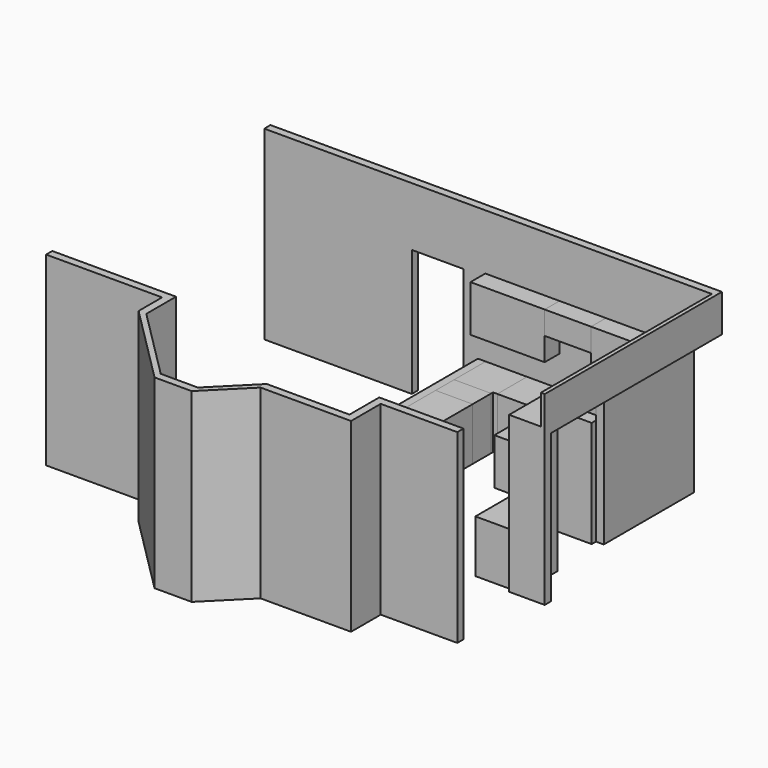
from build123d import *

# Parameters (mm, degrees)
F0_W      = 3556
F0_H      = 127
F1_DEPTH  = 3048
F3_DEPTH  = 3048
F4_W      = 127
F4_H      = 838.2
F5_DEPTH  = 3048
F6_W      = 1016
F6_H      = 127
F7_DEPTH  = 3048
F8_W      = 127
F8_H      = 482.6
F9_DEPTH  = 3048
F10_W     = 368.3
F10_H     = 127
F11_DEPTH = 3048
F12_W     = 996.95
F12_H     = 2095.5
F13_DEPTH = 25.4
F14_W     = 850.9
F14_H     = 965.2
F15_DEPTH = 127
F16_W     = 127
F16_H     = 965.2
F16_H_2   = 2082.8
F17_DEPTH = 2423.611736456
F18_W     = 1059.5979121052
F18_H     = 933.45
F19_DEPTH = 127
F21_W     = 457.2
F21_H     = 127
F22_DEPTH = 3048
F24_W     = 520.7
F24_H     = 3638.55
F25_DEPTH = 127
F26_W     = 3699.2286321938
F26_H     = 1626.0209083557
F27_DEPTH = 1270
F29_DEPTH = 127
F30_W     = 63.5
F30_H     = 615.95
F31_DEPTH = 3511.55
F32_W     = 685.8
F32_H     = 863.6
F33_DEPTH = 609.6
F34_W     = 685.8
F34_H     = 762
F35_DEPTH = 304.8
F36_W     = 901.7
F36_H     = 863.6
F37_DEPTH = 609.6
F38_W     = 825.5
F38_H     = 1752.6
F38_W_2   = 88.9
F39_DEPTH = 787.4
F40_W     = 609.6
F40_H     = 863.6
F41_DEPTH = 609.6
F45_DEPTH = 304.8
F46_W     = 1473.2
F46_H     = 2476.5
F47_DEPTH = 76.2
F48_W     = 914.4
F48_H     = 304.8
F49_DEPTH = 762
F50_W     = 762
F50_H     = 304.8
F51_DEPTH = 381
F52_W     = 1219.2
F52_H     = 304.8
F53_DEPTH = 762
F54_W     = 533.4
F54_H     = 609.6
F55_DEPTH = 863.6
F57_DEPTH = 863.6
F58_W     = 609.6
F58_H     = 381
F59_DEPTH = 863.6
F60_W     = 609.6
F60_H     = 990.6
F61_DEPTH = 863.6
F62_W     = 609.6
F62_H     = 127
F63_DEPTH = 863.6
F65_DEPTH = 863.6
F67_DEPTH = 863.6


with BuildPart() as f1:
    # F0 (on Top) → F1 (new body)
    with BuildSketch(Plane.XY):
        with Locations((-8.052283898, -253.0751817405)):
            Rectangle(F0_W, F0_H)
    extrude(amount=F1_DEPTH)

    # F2 (on face) → F3 (join, through all)
    with BuildSketch(Plane(origin=(0, 0, 0), x_dir=(1, 0, 0), z_dir=(0, 0, -1))):
        Polygon((1769.947716102, 2043.7751817405), (1769.947716102, 316.5751817405), (1769.947716102, 189.5751817405), (1896.947716102, 189.5751817405), (1896.947716102, 2043.7751817405), align=None)
    extrude(amount=-F3_DEPTH)

    # F14 (on face) → F15 (join, through all)
    with BuildSketch(Plane.XZ.offset(316.5751817405)):
        with Locations((-2211.502283898, 2565.4)):
            Rectangle(F14_W, F14_H)
    extrude(amount=-F15_DEPTH)

    # F16 (on face) → F17 (join, through all)
    with BuildSketch(Plane(origin=(-2636.952283898, 0, 0), x_dir=(0, -1, 0), z_dir=(-1, 0, 0))):
        with Locations((253.0751817405, 2565.4)):
            Rectangle(F16_W, F16_H)
        with Locations((253.0751817405, 1041.4)):
            Rectangle(F16_W, F16_H_2)
    extrude(amount=F17_DEPTH)



with BuildPart() as f5:
    # F4 (on face) → F5 (new body, through all)
    with BuildSketch(Plane(origin=(0, 0, 0), x_dir=(1, 0, 0), z_dir=(0, 0, -1))):
        with Locations((1833.447716102, 3409.0251817405)):
            Rectangle(F4_W, F4_H)
    extrude(amount=-F5_DEPTH)


with BuildPart() as f7:
    # F6 (on face) → F7 (new body, through all)
    with BuildSketch(Plane(origin=(0, 0, 0), x_dir=(1, 0, 0), z_dir=(0, 0, -1))):
        with Locations((1261.947716102, 5288.6251817405)):
            Rectangle(F6_W, F6_H)
    extrude(amount=-F7_DEPTH)

    # F8 (on face) → F9 (join, through all)
    with BuildSketch(Plane(origin=(0, 0, 0), x_dir=(1, 0, 0), z_dir=(0, 0, -1))):
        Polygon((-3028.564020354, 5277.9493022342), (-1843.1702123728, 6463.3431102153), (-1843.1702123728, 6590.3431102153), (-3155.564020354, 5277.9493022342), (-3155.564020354, 4795.3493022342), (-5060.564020354, 4795.3493022342), (-5060.564020354, 4668.3493022342), (-3028.564020354, 4668.3493022342), align=None)
        Polygon((-1233.5702123728, 6463.3431102153), (-604.952283898, 5834.7251817405), (-604.952283898, 5961.7251817405), (-1233.5702123728, 6590.3431102153), (-1843.1702123728, 6590.3431102153), (-1843.1702123728, 6463.3431102153), align=None)
        Polygon((-604.952283898, 5834.7251817405), (753.947716102, 5834.7251817405), (880.947716102, 5834.7251817405), (880.947716102, 5961.7251817405), (-604.952283898, 5961.7251817405), align=None)
        with Locations((817.447716102, 5593.4251817405)):
            Rectangle(F8_W, F8_H)
    extrude(amount=-F9_DEPTH)

    # F10 (on face) → F11 (join, through all)
    with BuildSketch(Plane(origin=(0, 0, 0), x_dir=(1, 0, 0), z_dir=(0, 0, -1))):
        with Locations((1954.097716102, 5288.6251817405)):
            Rectangle(F10_W, F10_H)
    extrude(amount=-F11_DEPTH)

    # F12 (on face) → F13 (join)
    with BuildSketch(Plane(origin=(0, -5225.1251817405, 0), x_dir=(-1, 0, 0), z_dir=(0, 1, 0))):
        with Locations((-1328.622716102, 1047.75)):
            Rectangle(F12_W, F12_H)
    extrude(amount=F13_DEPTH)

    # F46 (on face) → F47 (cut)
    with BuildSketch(Plane(origin=(-4153.2566612941, -4153.2566612941, 0), x_dir=(-0.7071067812, 0.7071067812, 0), z_dir=(0.7071067812, 0.7071067812, 0))):
        with Locations((-2428.7555863187, 1238.25)):
            Rectangle(F46_W, F46_H)
    extrude(amount=-F47_DEPTH, mode=Mode.SUBTRACT)


with BuildPart() as f1_1:
    add(f1.part)

    add(f5.part)  # F19 merges F5
    # F18 (on face) → F19 (join, through all)
    with BuildSketch(Plane(origin=(1769.947716102, 0, 0), x_dir=(0, -1, 0), z_dir=(-1, 0, 0))):
        with Locations((2573.5741377931, 2581.275)):
            Rectangle(F18_W, F18_H)
    extrude(amount=-F19_DEPTH)

    # F20: union 

    # F21 (on face) → F22 (join, through all)
    with BuildSketch(Plane.XY.offset(3048)):
        with Locations((2125.547716102, -3764.6251817405)):
            Rectangle(F21_W, F21_H)
    extrude(amount=-F22_DEPTH)

    # F24 (on offset) → F25 (join)
    with BuildSketch(Plane(origin=(0, 0, 2559.05), x_dir=(1, 0, 0), z_dir=(0, 0, -1))):
        with Locations((2030.297716102, 2008.8501817405)):
            Rectangle(F24_W, F24_H)
    extrude(amount=F25_DEPTH)

    # F26 (on face) → F27 (cut)
    with BuildSketch(Plane.YZ.offset(2290.647716102)):
        with Locations((-2166.1894978374, 3372.0604541779)):
            Rectangle(F26_W, F26_H)
    extrude(amount=-F27_DEPTH, mode=Mode.SUBTRACT)

    # F28 (on face) → F29 (join, through all)
    with BuildSketch(Plane(origin=(0, -189.5751817405, 0), x_dir=(-1, 0, 0), z_dir=(0, 1, 0))):
        Polygon((-1896.947716102, 2559.05), (-1896.947716102, 3048), (-2354.147716102, 3048), (-2354.147716102, 2432.05), (-2290.647716102, 2432.05), (-2290.647716102, 2559.05), align=None)
    extrude(amount=-F29_DEPTH)

    # F30 (on face) → F31 (join, through all)
    with BuildSketch(Plane(origin=(0, -189.5751817405, 0), x_dir=(-1, 0, 0), z_dir=(0, 1, 0))):
        with Locations((-2322.397716102, 2740.025)):
            Rectangle(F30_W, F30_H)
    extrude(amount=-F31_DEPTH)


with BuildPart() as f33:
    # F32 (on face) → F33 (new body)
    with BuildSketch(Plane(origin=(1769.947716102, 0, 0), x_dir=(0, -1, 0), z_dir=(-1, 0, 0))):
        with Locations((3415.3751817405, 431.8)):
            Rectangle(F32_W, F32_H)
    extrude(amount=F33_DEPTH)


with BuildPart() as f35:
    # F34 (on face) → F35 (new body)
    with BuildSketch(Plane(origin=(1769.947716102, 0, 0), x_dir=(0, -1, 0), z_dir=(-1, 0, 0))):
        with Locations((3406.3354730606, 1752.6)):
            Rectangle(F34_W, F34_H)
    extrude(amount=F35_DEPTH)


with BuildPart() as f37:
    # F36 (on face) → F37 (new body)
    with BuildSketch(Plane(origin=(1769.947716102, 0, 0), x_dir=(0, -1, 0), z_dir=(-1, 0, 0))):
        with Locations((767.4251817405, 431.8)):
            Rectangle(F36_W, F36_H)
    extrude(amount=F37_DEPTH)

    # F40 (on face) → F41 (join)
    with BuildSketch(Plane.XZ.offset(316.5751817405)):
        with Locations((855.547716102, 431.8)):
            Rectangle(F40_W, F40_H)
    extrude(amount=F41_DEPTH)


with BuildPart() as f39:
    # F38 (on face) → F39 (new body)
    with BuildSketch(Plane(origin=(1769.947716102, 0, 0), x_dir=(0, -1, 0), z_dir=(-1, 0, 0))):
        with Locations((1631.0251817405, 876.3)):
            Rectangle(F38_W, F38_H)
        with Locations((2088.2251817405, 876.3)):
            Rectangle(F38_W_2, F38_H)
    extrude(amount=F39_DEPTH)


with BuildPart() as f45:
    # F44 (on face) → F45 (new body, through all)
    with BuildSketch(Plane(origin=(1769.947716102, 0, 0), x_dir=(0, -1, 0), z_dir=(-1, 0, 0))):
        Polygon((2043.7751817405, 2114.55), (2043.7751817405, 2133.6), (316.5751817405, 2133.6), (316.5751817405, 1371.6), (1218.2751817405, 1371.6), (1218.2751817405, 1828.8), (2043.7751817405, 1828.8), align=None)
    extrude(amount=F45_DEPTH)

    # F48 (on face) → F49 (join, through all)
    with BuildSketch(Plane.XY.offset(2133.6)):
        with Locations((1007.947716102, -468.9751817405)):
            Rectangle(F48_W, F48_H)
    extrude(amount=-F49_DEPTH)


with BuildPart() as f51:
    # F50 (on face) → F51 (new body)
    with BuildSketch(Plane.XY.offset(2133.6)):
        with Locations((169.747716102, -468.9751817405)):
            Rectangle(F50_W, F50_H)
    extrude(amount=-F51_DEPTH)


with BuildPart() as f53:
    # F52 (on face) → F53 (new body, through all)
    with BuildSketch(Plane.XY.offset(2133.6)):
        with Locations((-820.852283898, -468.9751817405)):
            Rectangle(F52_W, F52_H)
    extrude(amount=-F53_DEPTH)


with BuildPart() as f55:
    # F54 (on face) → F55 (new body, through all)
    with BuildSketch(Plane.XY.offset(863.6)):
        with Locations((-477.952283898, -621.3751817405)):
            Rectangle(F54_W, F54_H)
    extrude(amount=-F55_DEPTH)


with BuildPart() as f57:
    # F56 (on face) → F57 (new body, through all)
    with BuildSketch(Plane.XY.offset(863.6)):
        Polygon((-814.502283898, -926.1751817405), (-744.652283898, -926.1751817405), (-744.652283898, -316.5751817405), (-1424.102283898, -316.5751817405), (-1424.102283898, -964.2751817405), (-814.502283898, -964.2751817405), align=None)
    extrude(amount=-F57_DEPTH)


with BuildPart() as f59:
    # F58 (on face) → F59 (new body, through all)
    with BuildSketch(Plane.XY.offset(863.6)):
        with Locations((-1119.302283898, -1154.7751817405)):
            Rectangle(F58_W, F58_H)
    extrude(amount=-F59_DEPTH)


with BuildPart() as f61:
    # F60 (on face) → F61 (new body, through all)
    with BuildSketch(Plane.XY.offset(863.6)):
        with Locations((-1119.302283898, -1840.5751817405)):
            Rectangle(F60_W, F60_H)
    extrude(amount=-F61_DEPTH)


with BuildPart() as f63:
    # F62 (on face) → F63 (new body, through all)
    with BuildSketch(Plane.XY.offset(863.6)):
        with Locations((-1119.302283898, -2399.3751817405)):
            Rectangle(F62_W, F62_H)
    extrude(amount=-F63_DEPTH)


with BuildPart() as f65:
    # F64 (on face) → F65 (new body, through all)
    with BuildSketch(Plane.XY.offset(863.6)):
        Polygon((-239.7658921496, -3037.6115734889), (-814.502283898, -2462.8751817405), (-1424.102283898, -2462.8751817405), (-1424.102283898, -2715.3797693631), (-670.8181859609, -3468.6638673002), align=None)
    extrude(amount=-F65_DEPTH)


with BuildPart() as f67:
    # F66 (on face) → F67 (new body, through all)
    with BuildSketch(Plane.XY.offset(863.6)):
        Polygon((-212.8251237863, -3010.6708051257), (-239.7658921496, -3037.6115734889), (-670.8181859609, -3468.6638673002), (-1424.102283898, -2715.3797693631), (-1424.102283898, -2462.8751817405), (-1424.102283898, -316.5751817405), (-1551.102283898, -316.5751817405), (-1551.102283898, -2767.9848917845), (-670.8181859609, -3648.2689897216), (-123.0225625757, -3100.4733663364), align=None)
    extrude(amount=-F67_DEPTH)


solid = Compound([f7.part, f1_1.part, f33.part, f35.part, f37.part, f39.part, f45.part, f51.part, f53.part, f55.part, f57.part, f59.part, f61.part, f63.part, f65.part, f67.part])
